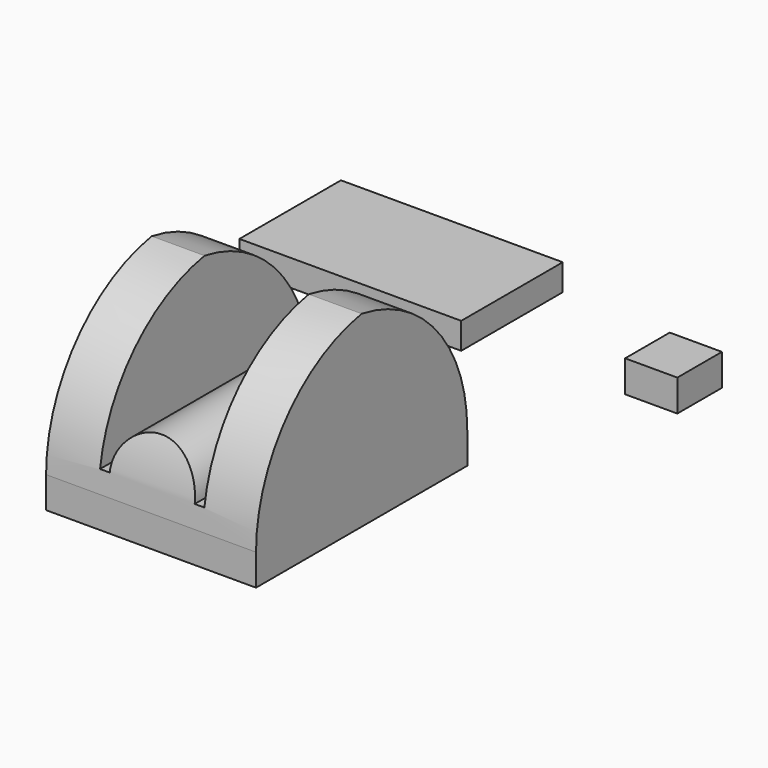
from build123d import *

# Parameters (mm, degrees)
F1_DEPTH    = 63.5
F2_T1_DEPTH = 203.2
F2_T3_DEPTH = 203.2
F5_W        = 53.3400033601
F5_H        = 30.5207520723
F6_DEPTH    = 6.35
F7_W        = 12.5505924225
F7_H        = 13.4063139558
F8_DEPTH    = 7.62


# Not quite as in the source:
# - a fillet or chamfer that OpenCascade refuses, or shapes differently, is made with other operations: its cross-section is extruded or revolved along the edge and cut away or added
# - the program builds the solid bodies; features that only make, move or delete a surface that nothing else refers to are left out


with BuildPart() as f1:
    # F0 (on Front) → F1 (new body)
    with BuildSketch(Plane.XZ):
        with BuildLine():
            Line((-25.2432132988, 0), (0, 0))
            Line((0, 0), (25.2432132988, 0))
            Line((25.2432132988, 0), (25.2432132988, 45.6259317593))
            Line((25.2432132988, 45.6259317593), (12.5432132988, 45.6259317593))
            Line((12.5432132988, 45.6259317593), (12.5432132988, 12.7))
            Line((12.5432132988, 12.7), (10.2199126405, 12.7))
            ThreePointArc((10.2199126405, 12.7), (0, 22.9199126405), (-10.2199126405, 12.7))
            Line((-10.2199126405, 12.7), (-12.5432132988, 12.7))
            Line((-12.5432132988, 12.7), (-12.5432132988, 45.6259317593))
            Line((-12.5432132988, 45.6259317593), (-25.2432132988, 45.6259317593))
            Line((-25.2432132988, 45.6259317593), (-25.2432132988, 0))
        make_face()
    extrude(amount=F1_DEPTH)

    # F2: fillet of radius 38.1 on 4 edges, made by hand

    # F2_s2 → F2_t1 (cut)
    with BuildSketch(Plane.YZ.offset(-120.4932132988)):
        with BuildLine():
            ThreePointArc((-25.4, 45.6259317593), (-52.3407683632, 34.4667001225), (-63.5, 7.5259317593))
            Line((-63.5, 7.5259317593), (-63.5, 45.6259317593))
            Line((-63.5, 45.6259317593), (-25.4, 45.6259317593))
        make_face()
        with BuildLine():
            ThreePointArc((0, 7.5259317593), (-11.1592316368, 34.4667001225), (-38.1, 45.6259317593))
            Line((-38.1, 45.6259317593), (0, 45.6259317593))
            Line((0, 45.6259317593), (0, 7.5259317593))
        make_face()
    extrude(amount=F2_T1_DEPTH, mode=Mode.SUBTRACT)

    # F2_s4 → F2_t3 (cut)
    with BuildSketch(Plane.YZ.offset(-82.7067867012)):
        with BuildLine():
            ThreePointArc((-25.4, 45.6259317593), (-52.3407683632, 34.4667001225), (-63.5, 7.5259317593))
            Line((-63.5, 7.5259317593), (-63.5, 45.6259317593))
            Line((-63.5, 45.6259317593), (-25.4, 45.6259317593))
        make_face()
        with BuildLine():
            ThreePointArc((0, 7.5259317593), (-11.1592316368, 34.4667001225), (-38.1, 45.6259317593))
            Line((-38.1, 45.6259317593), (0, 45.6259317593))
            Line((0, 45.6259317593), (0, 7.5259317593))
        make_face()
    extrude(amount=F2_T3_DEPTH, mode=Mode.SUBTRACT)


with BuildPart() as f6:
    # F5 (on Top) → F6 (new body)
    with BuildSketch(Plane.XY):
        with Locations((-31.5190923866, 51.0580763221)):
            Rectangle(F5_W, F5_H)
    extrude(amount=F6_DEPTH)


with BuildPart() as f8:
    # F7 (on Top) → F8 (new body)
    with BuildSketch(Plane.XY):
        with Locations((36.5108028054, 47.9204282165)):
            Rectangle(F7_W, F7_H)
    extrude(amount=F8_DEPTH)


solid = Compound([f1.part, f6.part, f8.part])
